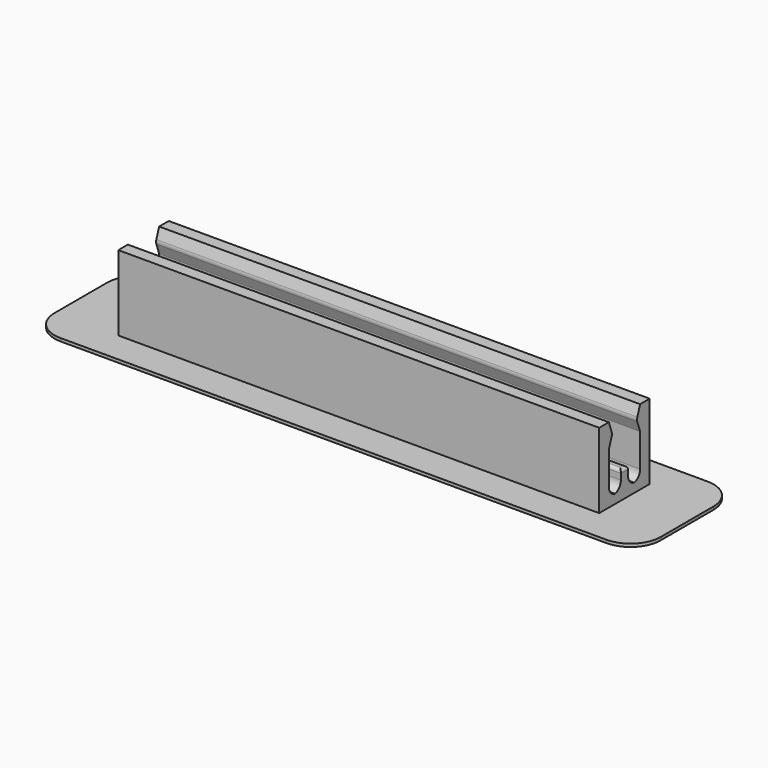
from build123d import *

# Parameters (mm, degrees)
F0_W        = 80
F0_H        = 6.5
F1_DEPTH    = 2
F0_H_2      = 2
F2_DEPTH    = 13
F3_W        = 1.5
F3_H        = 3
F4_DEPTH    = 80
F5_R        = 1
F6_R        = 1
F7_T1_DEPTH = 80
F8_R        = 0.5
F9_DEPTH    = 0.5


# Not quite as in the source:
# - a fillet or chamfer that OpenCascade refuses, or shapes differently, is made with other operations: its cross-section is extruded or revolved along the edge and cut away or added
# - a feature names something its author has since deleted; it is built from what else it names


with BuildPart() as f1:
    # F0 (on Top) → F1 (new body)
    with BuildSketch(Plane.XY):
        Rectangle(F0_W, F0_H)
    extrude(amount=F1_DEPTH)

    # F0 (on Top) → F2 (join)
    with BuildSketch(Plane.XY):
        with Locations((0, 4.25)):
            Rectangle(F0_W, F0_H_2)
        with Locations((0, -4.25)):
            Rectangle(F0_W, F0_H_2)
    extrude(amount=F2_DEPTH)

    # F3 (on face) → F4 (join)
    with BuildSketch(Plane(origin=(-40, 0, 0), x_dir=(0, -1, 0), z_dir=(-1, 0, 0))):
        Polygon((-3.25, 13), (-3.25, 9), (-2.55, 11), align=None)
        Polygon((2.55, 11), (3.25, 9), (3.25, 13), align=None)
        with Locations((0, 3.5)):
            Rectangle(F3_W, F3_H)
    extrude(amount=-F4_DEPTH)

    # F5
    f5_edges = [f1.edges().sort_by_distance(p)[0] for p in [
        (0, 2.55, 11),
    ]]
    fillet(f5_edges, radius=F5_R)

    # F6
    f6_edges = [f1.edges().sort_by_distance(p)[0] for p in [
        (0, -2.55, 11),
    ]]
    fillet(f6_edges, radius=F6_R)

    # F7: fillet of radius 1.5 on 4 edges, made by hand

    # F7_s2 → F7_t1 (join)
    with BuildSketch(Plane.YZ.offset(-40)):
        with BuildLine():
            ThreePointArc((-3.25, 3.5), (-2.8106601718, 2.4393398282), (-1.75, 2))
            Line((-1.75, 2), (-3.25, 2))
            Line((-3.25, 2), (-3.25, 3.5))
        make_face()
        with BuildLine():
            ThreePointArc((1.75, 2), (2.8106601718, 2.4393398282), (3.25, 3.5))
            Line((3.25, 3.5), (3.25, 2))
            Line((3.25, 2), (1.75, 2))
        make_face()
        with BuildLine():
            ThreePointArc((-2.25, 2), (-1.1893398282, 2.4393398282), (-0.75, 3.5))
            Line((-0.75, 3.5), (-0.75, 2))
            Line((-0.75, 2), (-2.25, 2))
        make_face()
        with BuildLine():
            ThreePointArc((0.75, 3.5), (1.1893398282, 2.4393398282), (2.25, 2))
            Line((2.25, 2), (0.75, 2))
            Line((0.75, 2), (0.75, 3.5))
        make_face()
    extrude(amount=F7_T1_DEPTH)

    # F8
    f8_edges = [f1.edges().sort_by_distance(p)[0] for p in [
        (0, -0.75, 5),
        (0, 0.75, 5),
        (-40, 0, 5),
        (40, 0, 5),
    ]]
    fillet(f8_edges, radius=F8_R)

    # F0 (on Top) → F9 (join)
    with BuildSketch(Plane.XY):
        with BuildLine():
            ThreePointArc((50.4157468677, 5.4975104332), (48.9512807736, 9.0330443391), (45.4157468677, 10.4975104332))
            Line((45.4157468677, 10.4975104332), (-45.4157468677, 10.4975104332))
            ThreePointArc((-45.4157468677, 10.4975104332), (-48.9512807736, 9.0330443391), (-50.4157468677, 5.4975104332))
            Line((-50.4157468677, 5.4975104332), (-50.4157468677, -5.4975104332))
            ThreePointArc((-50.4157468677, -5.4975104332), (-48.9512807736, -9.0330443391), (-45.4157468677, -10.4975104332))
            Line((-45.4157468677, -10.4975104332), (45.4157468677, -10.4975104332))
            ThreePointArc((45.4157468677, -10.4975104332), (48.9512807736, -9.0330443391), (50.4157468677, -5.4975104332))
            Line((50.4157468677, -5.4975104332), (50.4157468677, 5.4975104332))
        make_face()
        Polygon((-40, 5.25), (40, 5.25), (40, 3.25), (40, -3.25), (40, -5.25), (-40, -5.25), (-40, -3.25), (-40, 3.25), align=None, mode=Mode.SUBTRACT)
    extrude(amount=F9_DEPTH)


solid = f1.part
